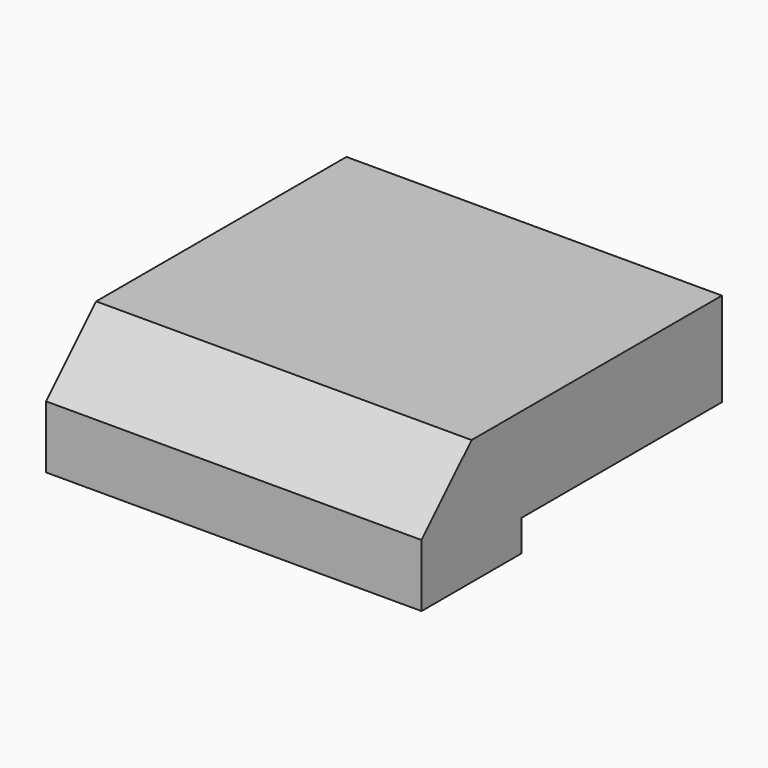
from build123d import *

# Parameters (mm, degrees)
F0_W     = 38.1
F0_H     = 38.1
F1_DEPTH = 9.525
F2_SIZE  = 6.35
F3_W     = 38.1
F3_H     = 12.7
F4_DEPTH = 3.175


# Not quite as in the source:
# - a feature of the source that left no trace in its solid (it failed there, or was rolled back) is left out


with BuildPart() as f1:
    # F0 (on Top) → F1 (new body)
    with BuildSketch(Plane.XY):
        Rectangle(F0_W, F0_H)
    extrude(amount=F1_DEPTH)

    # F2
    f2_edges = [f1.edges().sort_by_distance(p)[0] for p in [
        (0, -19.05, 9.525),
    ]]
    chamfer(f2_edges, length=F2_SIZE)

    # F3 (on face) → F4 (join)
    with BuildSketch(Plane(origin=(0, 0, 0), x_dir=(1, 0, 0), z_dir=(0, 0, -1))):
        with Locations((0, 12.7)):
            Rectangle(F3_W, F3_H)
    extrude(amount=F4_DEPTH)


solid = f1.part
